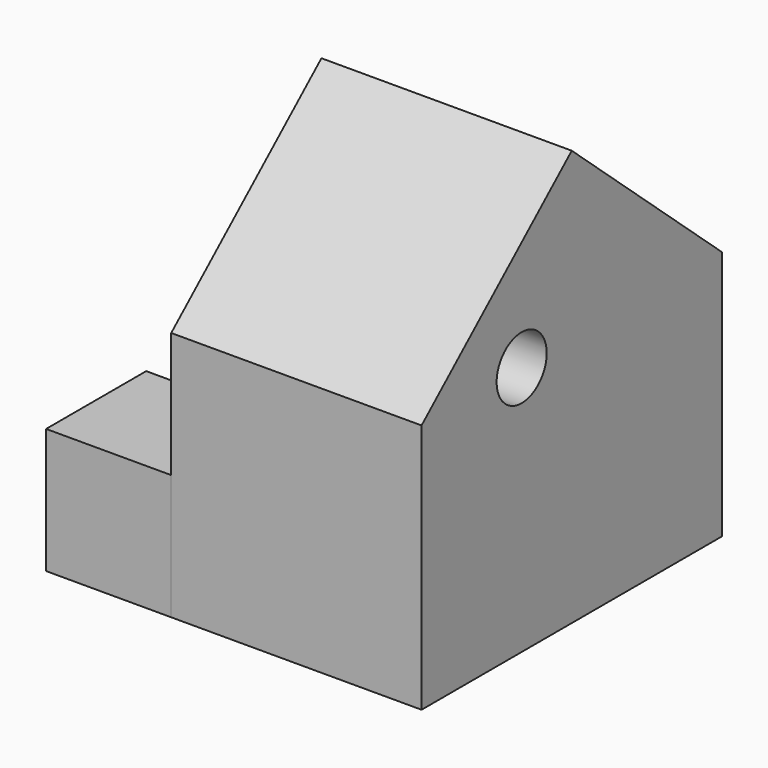
from build123d import *

# Parameters (mm, degrees)
F0_W     = 76.2
F0_H     = 50.8
F1_DEPTH = 50.8
F2_R     = 6.35
F3_DEPTH = 50.801
F5_DEPTH = 182
F6_W     = 25.4
F6_H     = 25.4
F7_DEPTH = 25.4


# Not quite as in the source:
# - an extrude ends at something that could not be found from the text; its depth is read off the source's solid


with BuildPart() as f1:
    # F0 (on Right) → F1 (new body)
    with BuildSketch(Plane.YZ):
        with Locations((-38.1, 25.4)):
            Rectangle(F0_W, F0_H)
        Polygon((-76.2, 50.8), (0, 50.8), (-38.1, 84.4010416505), align=None)
    extrude(amount=F1_DEPTH)

    # F2 (on face) → F3 (cut, through all)
    with BuildSketch(Plane.YZ.offset(50.8)):
        with Locations((-50.8, 50.8)):
            Circle(F2_R)
    extrude(amount=-F3_DEPTH, mode=Mode.SUBTRACT)

    # F4 (on Right) → F5 (cut, through all)
    with BuildSketch(Plane.YZ):
        with BuildLine():
            add(Edge.make_bspline(
                [(39.2249748279, 36.9491242033), (39.1707624624, 37.3291437229), (45.6123477048, 50.2146208478), (62.3111618585, 34.8878075899), (38.0564666464, 34.8735909417), (51.9023345065, 38.8834101985), (42.5172270712, 42.0337126477), (39.262733644, 36.6844412837), (39.2249748279, 36.9491242033)],
                knots=[0, 0, 0, 0, 0.1947455978, 0.3915991224, 0.5908148595, 0.7271841262, 0.8643600374, 1, 1, 1, 1], degree=3))
        make_face()
    extrude(amount=-F5_DEPTH, mode=Mode.SUBTRACT)


with BuildPart() as f7:
    # F6 (on face) → F7 (new body)
    with BuildSketch(Plane(origin=(0, 0, 0), x_dir=(0, -1, 0), z_dir=(-1, 0, 0))):
        with Locations((63.5, 12.7)):
            Rectangle(F6_W, F6_H)
    extrude(amount=F7_DEPTH)


solid = Compound([f1.part, f7.part])
